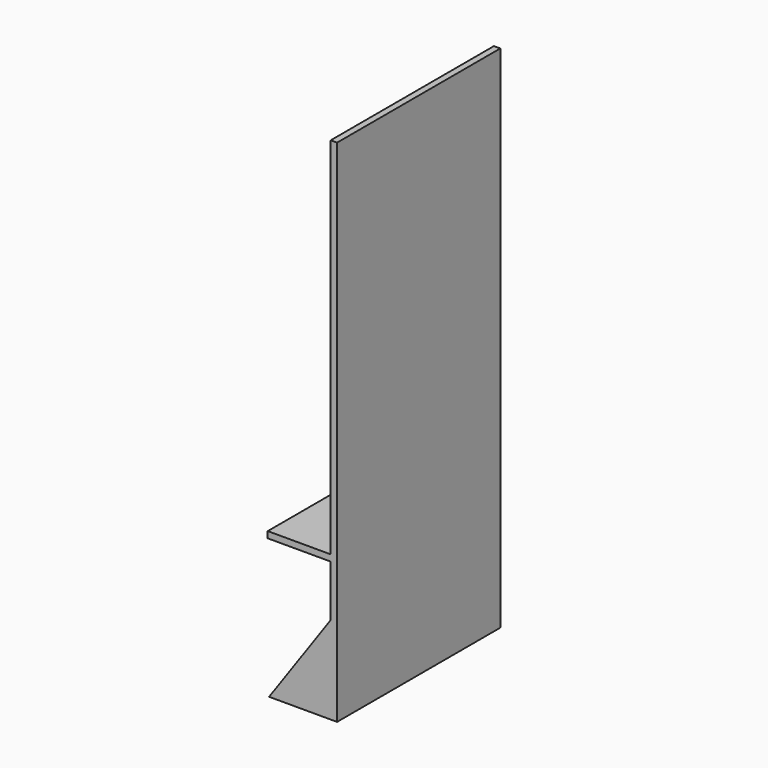
from build123d import *

# Parameters (mm, degrees)
F1_DEPTH = 19.05
F2_DEPTH = 609.6
F3_E0_W  = 1524
F3_E0_H  = 609.6
F4_DEPTH = 19.05
F5_DEPTH = 25.4
F6_E4_W  = 207.3184425354
F6_E4_H  = 609.6
F7_DEPTH = 19.05


with BuildPart() as f1:
    # F0 (on Front) → F1 (new body)
    with BuildSketch(Plane.XZ):
        Polygon((-24.7226779938, -763.8654754907), (-24.7226779938, -474.9317169189), (-227.9226779938, -763.8654754907), align=None)
    extrude(amount=F1_DEPTH)

    # F0 (on Front) → F2 (join)
    with BuildSketch(Plane.XZ):
        Polygon((-24.7226779938, -763.8654754907), (-24.7226779938, -474.9317169189), (-227.9226779938, -763.8654754907), align=None)
    extrude(amount=F2_DEPTH)

    # F3_E0 (on explicit) → F4 (join)
    with BuildSketch(Plane(origin=(-24.7226779938, 0, 760.1345245093), x_dir=(0, 0, -1), z_dir=(-1, 0, 0))):
        with Locations((762, 304.8)):
            Rectangle(F3_E0_W, F3_E0_H)
    extrude(amount=F4_DEPTH)

    # F0 (on Front) → F5 (join)
    with BuildSketch(Plane.XZ):
        Polygon((-24.7226779938, -763.8654754907), (-24.7226779938, -474.9317169189), (-227.9226779938, -763.8654754907), align=None)
    extrude(amount=F5_DEPTH)

    # F6_E4 (on explicit) → F7 (join)
    with BuildSketch(Plane(origin=(-24.7226779938, 0, -348.2956886292), x_dir=(-1, 0, 0), z_dir=(0, 0, 1))):
        with Locations((103.6592212677, 304.8)):
            Rectangle(F6_E4_W, F6_E4_H)
    extrude(amount=F7_DEPTH)


solid = f1.part
